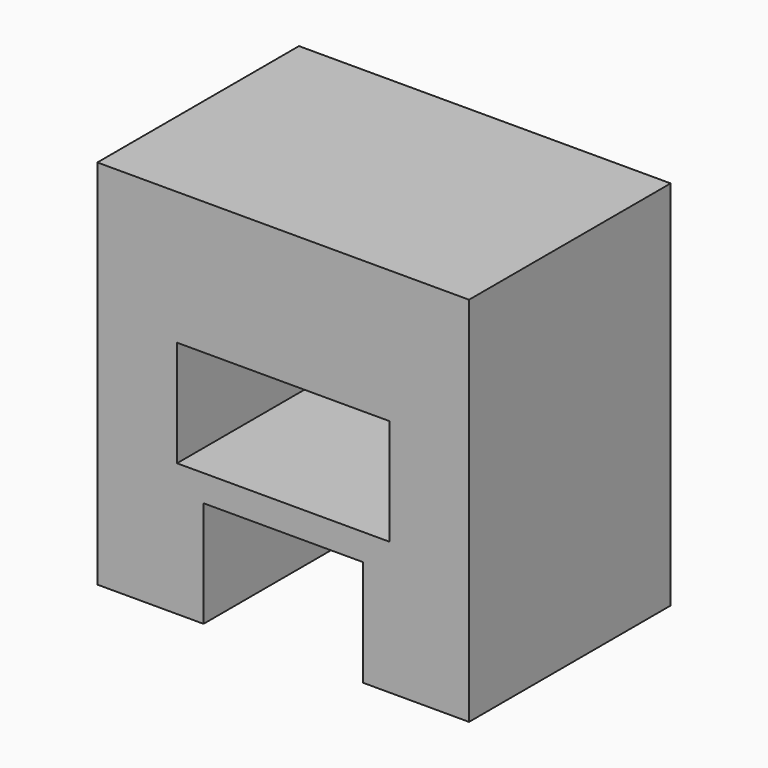
from build123d import *

# Parameters (mm, degrees)
F1_DEPTH = 500
F3_DEPTH = 25.4
F4_W     = 400
F4_H     = 200
F5_DEPTH = 474.601


# Not quite as in the source:
# - a feature names something its author has since deleted; it is built from what else it names


with BuildPart() as f1:
    # F0 (on Front) → F1 (new body)
    with BuildSketch(Plane.XZ):
        Polygon((350, -350), (350, 350), (-350, 350), (-350, -350), (-150, -350), (-150, -150), (150, -150), (150, -350), align=None)
    extrude(amount=F1_DEPTH)

    # F3 (cut): a face of the model
    f3_faces = [f1.faces().sort_by_distance(p)[0] for p in [
        (0, 0, 34.8837209302),
    ]]
    extrude(f3_faces, amount=-F3_DEPTH, mode=Mode.SUBTRACT)

    # F4 (on face) → F5 (cut, through all)
    with BuildSketch(Plane.XZ.offset(500)):
        Rectangle(F4_W, F4_H)
    extrude(amount=-F5_DEPTH, mode=Mode.SUBTRACT)


solid = f1.part
